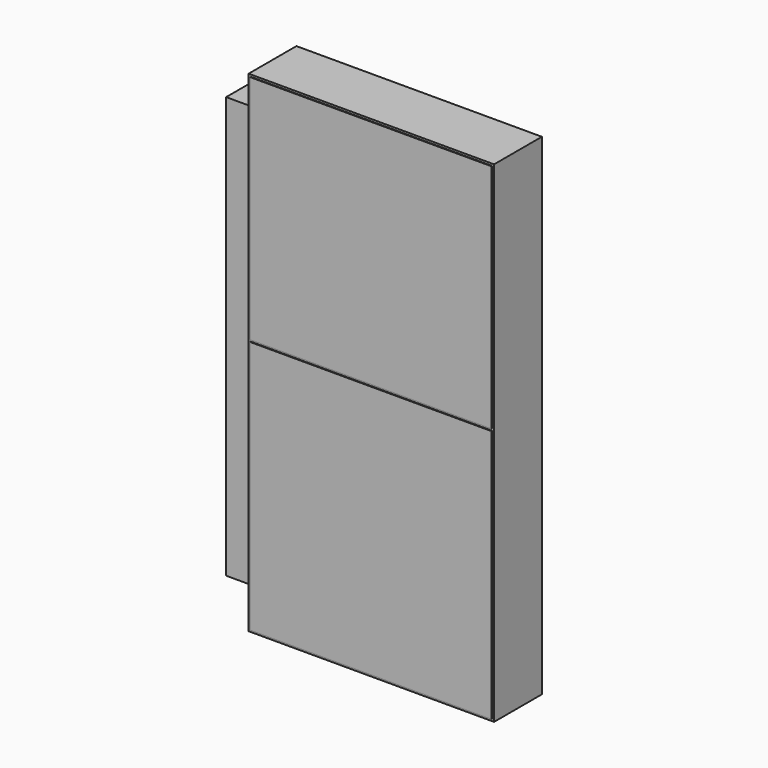
from build123d import *

# Parameters (mm, degrees)
F0_W     = 600
F0_H     = 1200
F1_DEPTH = 75
F2_W     = 600
F2_H     = 1200
F2_W_2   = 590
F2_H_2   = 620
F2_H_3   = 565
F3_DEPTH = 2
F4_W     = 96
F4_H     = 1030
F5_DEPTH = 75


# Not quite as in the source:
# - a pattern or mirror of a feature is missing from the dataset's text; its kind, count and spacing are read off the source's solid


with BuildPart() as f1:
    # F0 (on Front) → F1 (new body, symmetric)
    with BuildSketch(Plane.XZ):
        with Locations((-546.9189941883, 533.8190406561)):
            Rectangle(F0_W, F0_H)
    extrude(amount=F1_DEPTH, both=True)

    # F2 (on face) → F3 (cut)
    with BuildSketch(Plane.XZ.offset(75)):
        with Locations((-546.9189941883, 533.8190406561)):
            Rectangle(F2_W, F2_H)
        with Locations((-546.9189941883, 248.8190406561)):
            Rectangle(F2_W_2, F2_H_2, mode=Mode.SUBTRACT)
        with Locations((-546.9189941883, 846.3190406561)):
            Rectangle(F2_W_2, F2_H_3, mode=Mode.SUBTRACT)
    f3 = extrude(amount=-F3_DEPTH, mode=Mode.SUBTRACT)

    # F3_copies: F3 across plane
    add(f3.mirror(Plane.ZX), mode=Mode.SUBTRACT)

    # F4 (on face) → F5 (join)
    with BuildSketch(Plane(origin=(-846.9189941883, 0, 0), x_dir=(0, -1, 0), z_dir=(-1, 0, 0))):
        with Locations((0, 533.8190406561)):
            Rectangle(F4_W, F4_H)
    extrude(amount=F5_DEPTH)


solid = f1.part
